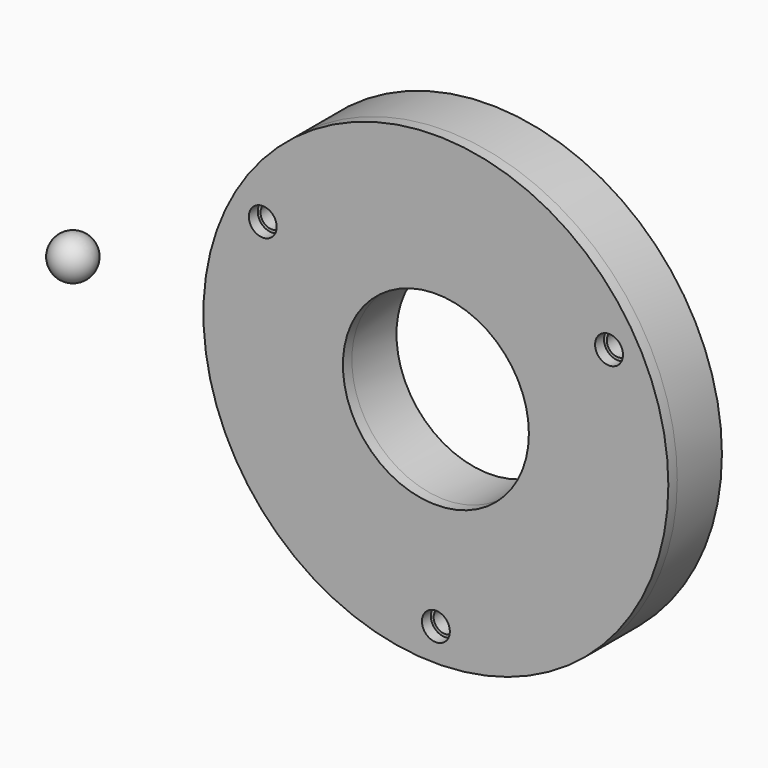
from build123d import *

# Parameters (mm, degrees)
F0_R            = 25
F0_R_2          = 10
F1_DEPTH        = 6
F3_DEPTH        = 4.7
F3_COPIES_COUNT = 3
F5_D            = 2.4
F5_COPIES_COUNT = 3
F6_R            = 25
F6_R_2          = 1.5
F6_R_3          = 10
F7_DEPTH        = 1.2


# Not quite as in the source:
# - a pattern or mirror of a feature is missing from the dataset's text; its kind, count and spacing are read off the source's solid


with BuildPart() as f1:
    # F0 (on Front) → F1 (new body)
    with BuildSketch(Plane.XZ):
        Circle(F0_R)
        Circle(F0_R_2, mode=Mode.SUBTRACT)
    extrude(amount=-F1_DEPTH)

    # F2 (on face) → F3 (cut)
    with BuildSketch(Plane.XZ):
        with BuildLine():
            ThreePointArc((-16.2634559673, 16.2634559673), (-16.2634559673, 12.7279220614), (-12.7279220614, 12.7279220614))
            ThreePointArc((-12.7279220614, 12.7279220614), (0, 18), (12.7279220614, 12.7279220614))
            ThreePointArc((12.7279220614, 12.7279220614), (16.2634559673, 12.7279220614), (16.2634559673, 16.2634559673))
            ThreePointArc((16.2634559673, 16.2634559673), (0, 23), (-16.2634559673, 16.2634559673))
        make_face()
    f3 = extrude(amount=-F3_DEPTH, mode=Mode.SUBTRACT)

    # F3_copies: F3 ×3 about axis
    f3_copies_axis = Axis((0, 0, 0), (0, 1, 0))
    for i in range(1, F3_COPIES_COUNT):
        add(f3.rotate(f3_copies_axis, i * 360 / F3_COPIES_COUNT), mode=Mode.SUBTRACT)

    # F5 (through all)
    with Locations(Plane.XZ):
        with Locations((0, -21.5)):
            f5 = Hole(F5_D / 2)

    # F5_copies: F5 ×3 about axis
    f5_copies_axis = Axis((0, 0, 0), (0, 1, 0))
    for i in range(1, F5_COPIES_COUNT):
        add(f5.rotate(f5_copies_axis, i * 360 / F5_COPIES_COUNT), mode=Mode.SUBTRACT)


with BuildPart() as f7:
    # F6 (on face) → F7 (new body)
    with BuildSketch(Plane.XZ):
        Circle(F6_R)
        with Locations((0, -21.5)):
            Circle(F6_R_2, mode=Mode.SUBTRACT)
        with Locations((-18.6195461814, 10.75)):
            Circle(F6_R_2, mode=Mode.SUBTRACT)
        Circle(F6_R_3, mode=Mode.SUBTRACT)
        with Locations((18.6195461814, 10.75)):
            Circle(F6_R_2, mode=Mode.SUBTRACT)
    extrude(amount=F7_DEPTH)


with BuildPart() as f9:
    # F8 (on Front) → F9 (revolve)
    with BuildSketch(Plane.XZ):
        with BuildLine():
            Line((-42.25, 0), (-37.75, 0))
            ThreePointArc((-37.75, 0), (-40, 2.25), (-42.25, 0))
        make_face()
    revolve(axis=Axis((-40, 0, 0), (1, 0, 0)))


solid = Compound([f1.part, f7.part, f9.part])
